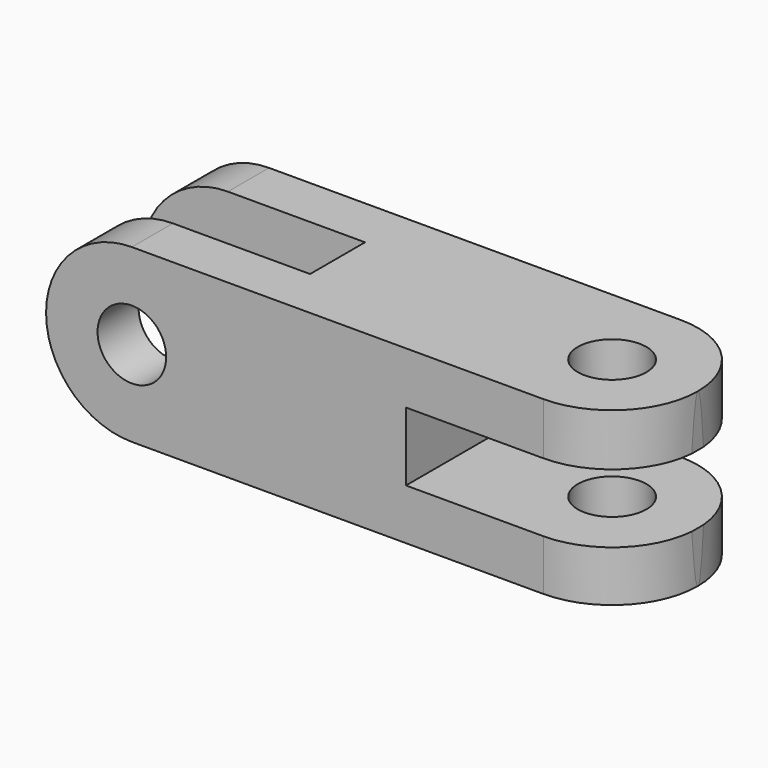
from build123d import *

# Parameters (mm, degrees)
F0_R     = 6.35
F1_DEPTH = 31.75
F3_DEPTH = 31.751


with BuildPart() as f1:
    # F0 (on Front) → F1 (new body)
    with BuildSketch(Plane.XZ):
        with BuildLine():
            Line((53.7298298755, 11.3510093242), (-38.3451701245, 11.3510093242))
            ThreePointArc((-38.3451701245, 11.3510093242), (-54.2201701245, -4.5239906758), (-38.3451701245, -20.3989906758))
            Line((-38.3451701245, -20.3989906758), (53.7298298755, -20.3989906758))
            Line((53.7298298755, -20.3989906758), (53.6711269855, -10.9930955659))
            Line((53.6711269855, -10.9930955659), (12.3961269855, -10.9930955659))
            Line((12.3961269855, -10.9930955659), (12.3961269855, 1.7069044341))
            Line((12.3961269855, 1.7069044341), (53.6711269855, 1.7069044341))
            Line((53.6711269855, 1.7069044341), (53.7298298755, 11.3510093242))
        make_face()
        with Locations((-38.3451701245, -4.5239906758)):
            Circle(F0_R, mode=Mode.SUBTRACT)
    extrude(amount=F1_DEPTH)

    # F2 (on face) → F3 (cut, through all)
    with BuildSketch(Plane.XY.offset(11.3510093242)):
        with BuildLine():
            Line((53.7298298755, 0), (37.8548298755, 0))
            ThreePointArc((37.8548298755, 0), (49.0801500268, -4.6496798487), (53.7298298755, -15.875))
            Line((53.7298298755, -15.875), (53.7298298755, 0))
        make_face()
        with BuildLine():
            Line((53.7298298755, -31.75), (53.7298298755, -15.875))
            ThreePointArc((53.7298298755, -15.875), (49.0801500268, -27.1003201513), (37.8548298755, -31.75))
            Line((37.8548298755, -31.75), (53.7298298755, -31.75))
        make_face()
        Polygon((-38.3451701245, -22.2507314071), (-38.3451701245, -9.525), (-54.2339347303, -9.525), (-54.2339347303, -22.2551717675), align=None)
        Polygon((-12.9589347303, -9.525), (-38.3451701245, -9.525), (-38.3451701245, -22.2507314071), (-12.9589347303, -22.243636832), align=None)
        with BuildLine():
            ThreePointArc((37.8548298755, -22.225), (42.344957936, -20.3651280605), (44.2048298755, -15.875))
            ThreePointArc((44.2048298755, -15.875), (33.3647018149, -11.3848719395), (37.8548298755, -22.225))
        make_face()
    extrude(amount=-F3_DEPTH, mode=Mode.SUBTRACT)


solid = f1.part
